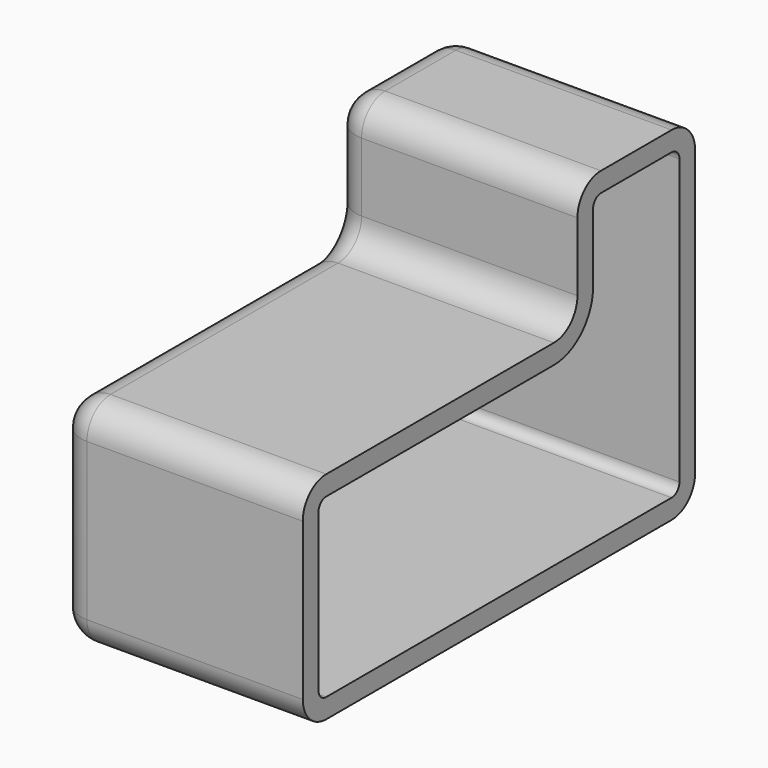
from build123d import *

# Parameters (mm, degrees)
F1_DEPTH = 25
F2_F1_R  = 3
F2_F2_R  = 3
F3_T     = -2


with BuildPart() as f1:
    # F0 (on Right) → F1 (new body)
    with BuildSketch(Plane.YZ):
        Polygon((0, 27.4222218948), (0, 14.4222218948), (-35, 14.4222218948), (-35, -7.5777781052), (15, -7.5777781052), (15, 27.4222218948), align=None)
    extrude(amount=F1_DEPTH)

    # F2: fillet of radius 3 on 11 edges, made by hand

    # F2_f1
    f2_f1_edges = [f1.edges().sort_by_distance(p)[0] for p in [
        (12.5, 0, 14.4222218948),
    ]]
    fillet(f2_f1_edges, radius=F2_F1_R)

    # F2_f2
    f2_f2_edges = [f1.edges().sort_by_distance(p)[0] for p in [
        (0, -10, -7.5777781052),
        (0, -35, 3.4222218948),
        (0, -19, 14.4222218948),
        (0, 7.5, 27.4222218948),
        (0, 15, 9.9222218948),
        (12.5, 15, -7.5777781052),
        (12.5, -35, -7.5777781052),
        (12.5, -35, 14.4222218948),
        (12.5, 0, 27.4222218948),
        (12.5, 15, 27.4222218948),
        (0, -0.8786796564, 15.3009015512),
    ]]
    fillet(f2_f2_edges, radius=F2_F2_R)

    # F3
    f3_openings = [f1.faces().sort_by_distance(p)[0] for p in [
        (25, -7.351061, 6.036173),
    ]]
    offset(amount=F3_T, openings=f3_openings)


solid = f1.part
